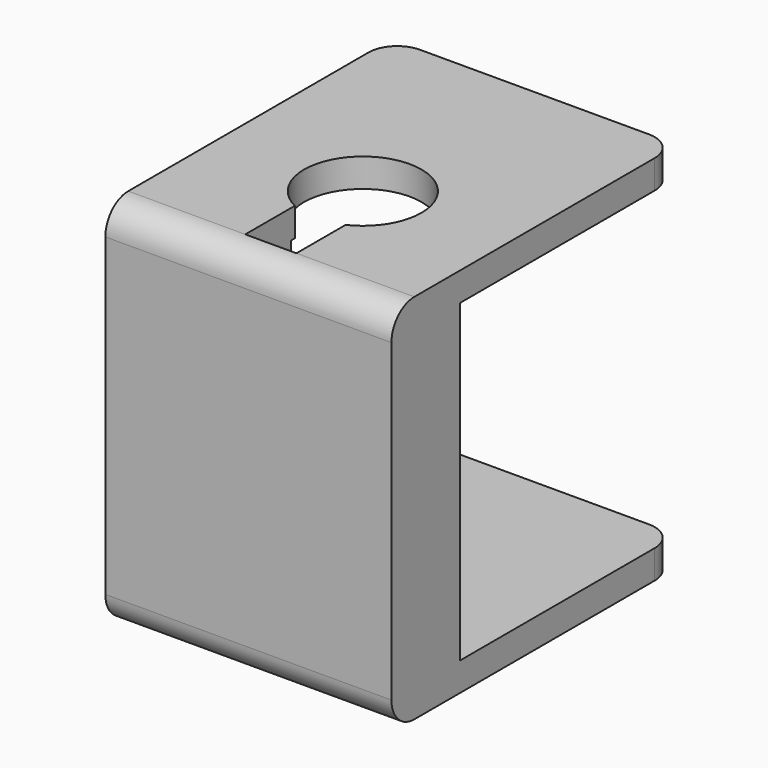
from build123d import *

# Parameters (mm, degrees)
F0_W     = 4
F0_H     = 18
F1_DEPTH = 20
F3_DEPTH = 30
F5_DEPTH = 4
F6_R     = 1.99999


# Not quite as in the source:
# - a fillet or chamfer is up to 0.001 mm smaller than in the source, because OpenCascade refuses the exact size
# - a feature names something its author has since deleted; it is built from what else it names


with BuildPart() as f1:
    # F0 (on Right) → F1 (new body)
    with BuildSketch(Plane.YZ):
        Polygon((0, 26), (0, 0), (25, 0), (25, 2), (6, 2), (6, 4), (2, 4), (2, 22), (6, 22), (6, 24), (25, 24), (25, 26), align=None)
        with Locations((4, 13)):
            Rectangle(F0_W, F0_H)
    extrude(amount=F1_DEPTH)

    # F2 (on face) → F3 (cut)
    with BuildSketch(Plane.XY.offset(26)):
        with BuildLine():
            ThreePointArc((11.7568019778, 6.295455924), (9.9657604027, 5.900142972), (8.1815710291, 6.3253141525))
            Line((8.1815710291, 6.3253141525), (8.1815710291, 2))
            Line((8.1815710291, 2), (10, 2))
            Line((10, 2), (11.7568019778, 2))
            Line((11.7568019778, 2), (11.7568019778, 6.295455924))
        make_face()
        with BuildLine():
            ThreePointArc((11.7568019778, 6.295455924), (13.4650316094, 7.8082983904), (14.1, 10))
            ThreePointArc((14.1, 10), (7.8373117169, 13.4832139455), (8.1815710291, 6.3253141525))
            ThreePointArc((8.1815710291, 6.3253141525), (9.9657604027, 5.900142972), (11.7568019778, 6.295455924))
        make_face()
    extrude(amount=-F3_DEPTH, mode=Mode.SUBTRACT)

    # F4 (on face) → F5 (join)
    with BuildSketch(Plane(origin=(0, 2, 0), x_dir=(-1, 0, 0), z_dir=(0, 1, 0))):
        with BuildLine():
            ThreePointArc((-11.7568019778, 12), (-11.0496951966, 12.2928932188), (-10.7568019778, 13))
            ThreePointArc((-10.7568019778, 13), (-11.0496951966, 13.7071067812), (-11.7568019778, 14))
            Line((-11.7568019778, 14), (-11.7568019778, 12))
        make_face()
        with BuildLine():
            Line((-8.1815710291, 18), (-8.1815710291, 20))
            ThreePointArc((-8.1815710291, 20), (-9.1815710291, 19), (-8.1815710291, 18))
        make_face()
        with BuildLine():
            ThreePointArc((-7.1815710291, 19), (-7.4744642479, 19.7071067812), (-8.1815710291, 20))
            Line((-8.1815710291, 20), (-8.1815710291, 18))
            ThreePointArc((-8.1815710291, 18), (-7.4744642479, 18.2928932188), (-7.1815710291, 19))
        make_face()
        with BuildLine():
            ThreePointArc((-8.1815710291, 8), (-9.1815710291, 7), (-8.1815710291, 6))
            Line((-8.1815710291, 6), (-8.1815710291, 8))
        make_face()
    extrude(amount=F5_DEPTH)

    # F6 (radius 2 in the source; OpenCascade refuses exactly that, so slightly less here)
    f6_edges = [f1.edges().sort_by_distance(p)[0] for p in [
        (10, 0, 26),
        (10, 0, 0),
        (20, 25, 1),
        (0, 25, 1),
        (0, 25, 25),
        (20, 25, 25),
    ]]
    fillet(f6_edges, radius=F6_R)


solid = f1.part
